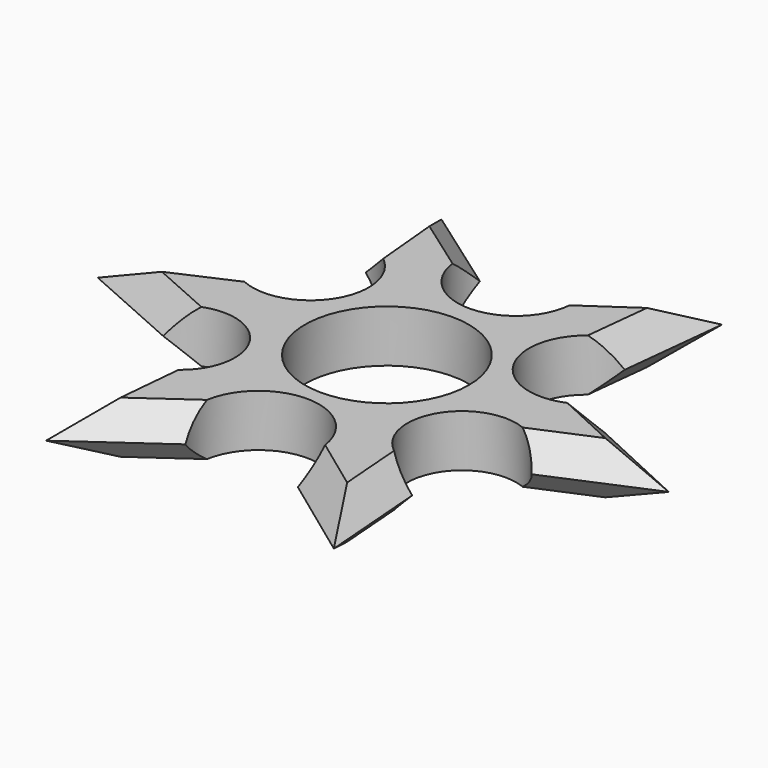
from build123d import *

# Parameters (mm, degrees)
F0_R         = 11
F1_DEPTH     = 7
F2_SIZE      = 3.81
F3_T1_DEPTH  = 34.6394313852
F3_T3_DEPTH  = 34.3439110976
F4_SIZE      = 3.81
F5_T1_DEPTH  = 35.2279158768
F5_T3_DEPTH  = 35.1515641575
F5_T5_DEPTH  = 34.8076073963
F5_T7_DEPTH  = 34.8076073963
F5_T9_DEPTH  = 34.5979192148
F5_T11_DEPTH = 35.1515641575
F5_T13_DEPTH = 35.2279158768
F5_T15_DEPTH = 34.6394313852
F5_T17_DEPTH = 34.8076073963
F6_T1_DEPTH  = 29.7856896268


# Not quite as in the source:
# - a fillet or chamfer that OpenCascade refuses, or shapes differently, is made with other operations: its cross-section is extruded or revolved along the edge and cut away or added


with BuildPart() as f1:
    # F0 (on Top) → F1 (new body)
    with BuildSketch(Plane.XY):
        with BuildLine():
            Line((-19.3098304855, 33.4750442975), (-17.9191186068, 18.4962593726))
            ThreePointArc((-17.9191186068, 18.4962593726), (-12.1734101316, 6.7065768921), (-25.2838117957, 6.35))
            Line((-25.2838117957, 6.35), (-39.5676235915, 0))
            Line((-39.5676235915, 0), (-25.3535799067, -6.3189839441))
            ThreePointArc((-25.3535799067, -6.3189839441), (-12.9763127609, -6.8724869317), (-18.8926645602, -17.7582523592))
            Line((-18.8926645602, -17.7582523592), (-20.2989239466, -32.9044930863))
            Line((-20.2989239466, -32.9044930863), (-7.891724267, -24.1040629982))
            ThreePointArc((-7.891724267, -24.1040629982), (-0.2207247048, -12.9944902326), (7.1436805269, -24.3096295115))
            Line((7.1436805269, -24.3096295115), (19.2464965418, -33.1737534264))
            Line((19.2464965418, -33.1737534264), (19.2872961226, -33.1740312262))
            Line((19.2872961226, -33.1740312262), (18.113880894, -18.0395493303))
            ThreePointArc((18.113880894, -18.0395493303), (12.3636945983, -7.0651033251), (24.7479456966, -6.6998194754))
            Line((24.7479456966, -6.6998194754), (39.056406052, -0.5976429607))
            Line((39.056406052, -0.5976429607), (24.8707754105, 5.9687611329))
            ThreePointArc((24.8707754105, 5.9687611329), (11.7673092468, 6.524596873), (17.6915767021, 18.225572644))
            Line((17.6915767021, 18.225572644), (19.3098304855, 33.1814855899))
            Line((19.3098304855, 33.1814855899), (7.1525325905, 24.8331700857))
            ThreePointArc((7.1525325905, 24.8331700857), (0.2505296838, 13.6219778067), (-6.9026308059, 24.6746142094))
            Line((-6.9026308059, 24.6746142094), (-19.3098304855, 33.4750442975))
        make_face()
        Circle(F0_R, mode=Mode.SUBTRACT)
    extrude(amount=F1_DEPTH)

    # F2
    f2_edges = [f1.edges().sort_by_distance(p)[0] for p in [
        (18.500704, 25.703529, 7),
        (13.231182, 29.007328, 7),
    ]]
    chamfer(f2_edges, length=F2_SIZE)

    # F3: chamfer of 3.81 on 2 edges, made by hand

    # F3_s2 → F3_t1 (cut)
    with BuildSketch(Plane(origin=(1.0999249917, 10.1655145758, 0), x_dir=(0, 0, 1), z_dir=(0.1075737229, 0.9941971103, 0))):
        Polygon((3.81, 15.6283217323), (0, 11.8183217323), (0, 15.6283217323), align=None)
    extrude(amount=F3_T1_DEPTH, mode=Mode.SUBTRACT)

    # F3_s4 → F3_t3 (cut)
    with BuildSketch(Plane(origin=(36.6832724438, 25.190098551, 0), x_dir=(0, 0, 1), z_dir=(-0.8243528709, -0.5660762706, 0))):
        Polygon((0, 12.6124160802), (3.81, 16.4224160802), (0, 16.4224160802), align=None)
    extrude(amount=F3_T3_DEPTH, mode=Mode.SUBTRACT)

    # F4 (call 1 of 6: OpenCascade refuses the feature's edges together)
    f4_edges = [f1.edges().sort_by_distance(p)[0] for p in [
        (31.902176, -3.648731, 7),
        (31.963591, 2.685559, 7),
    ]]
    chamfer(f4_edges, length=F4_SIZE)

    # F4#2 (call 2 of 6)
    f4_2_edges = [f1.edges().sort_by_distance(p)[0] for p in [
        (18.700589, -25.60679, 7),
    ]]
    chamfer(f4_2_edges, length=F4_SIZE)

    # F4#3 (call 3 of 6)
    f4_3_edges = [f1.edges().sort_by_distance(p)[0] for p in [
        (13.195089, -28.741691, 7),
    ]]
    chamfer(f4_3_edges, length=F4_SIZE)

    # F4#4 (call 4 of 6)
    f4_4_edges = [f1.edges().sort_by_distance(p)[0] for p in [
        (-14.095324, -28.504278, 7),
        (-19.595794, -25.331373, 7),
    ]]
    chamfer(f4_4_edges, length=F4_SIZE)

    # F4#5 (call 5 of 6)
    f4_5_edges = [f1.edges().sort_by_distance(p)[0] for p in [
        (-32.460602, -3.159492, 7),
        (-32.425718, 3.175, 7),
    ]]
    chamfer(f4_5_edges, length=F4_SIZE)

    # F4#6 (call 6 of 6)
    f4_6_edges = [f1.edges().sort_by_distance(p)[0] for p in [
        (-18.614475, 25.985652, 7),
        (-13.106231, 29.074829, 7),
    ]]
    chamfer(f4_6_edges, length=F4_SIZE)

    # F5: chamfer of 3.81 on 9 edges, made by hand

    # F5_s2 → F5_t1 (cut)
    with BuildSketch(Plane(origin=(41.2840936669, -19.1100451228, 0), x_dir=(0, 0, 1), z_dir=(-0.9074917218, 0.4200699643, 0))):
        Polygon((0, 12.0540670557), (3.81, 15.8640670557), (0, 15.8640670557), align=None)
    extrude(amount=F5_T1_DEPTH, mode=Mode.SUBTRACT)

    # F5_s4 → F5_t3 (cut)
    with BuildSketch(Plane(origin=(9.5091795604, 4.0554113263, 0), x_dir=(0, 0, 1), z_dir=(0.9198423531, 0.3922882173, 0))):
        Polygon((0, 12.0611052097), (3.81, 15.8711052097), (0, 15.8711052097), align=None)
    extrude(amount=F5_T3_DEPTH, mode=Mode.SUBTRACT)

    # F5_s6 → F5_t5 (cut)
    with BuildSketch(Plane(origin=(-37.0237803275, -26.260977399, 0), x_dir=(0, 0, 1), z_dir=(0.8156523083, 0.5785424029, 0))):
        Polygon((0, 11.2848375041), (3.81, 15.0948375041), (0, 15.0948375041), align=None)
    extrude(amount=F5_T5_DEPTH, mode=Mode.SUBTRACT)

    # F5_s8 → F5_t7 (cut)
    with BuildSketch(Plane(origin=(-0.8903351992, -9.5894337742, 0), x_dir=(0, 0, 1), z_dir=(-0.0924478322, -0.9957175294, 0))):
        Polygon((0, 13.3600453443), (3.81, 17.1700453443), (0, 17.1700453443), align=None)
    extrude(amount=F5_T7_DEPTH, mode=Mode.SUBTRACT)

    # F5_s10 → F5_t9 (cut)
    with BuildSketch(Plane(origin=(8.3331341524, -6.1032022329, 0), x_dir=(0, 0, 1), z_dir=(0.806763245, -0.5908748315, 0))):
        Polygon((0, 11.5810945617), (3.81, 15.3910945617), (0, 15.3910945617), align=None)
    extrude(amount=F5_T9_DEPTH, mode=Mode.SUBTRACT)

    # F5_s12 → F5_t11 (cut)
    with BuildSketch(Plane(origin=(-41.9914373351, 18.6676799506, 0), x_dir=(0, 0, 1), z_dir=(0.9137726258, -0.406226031, 0))):
        Polygon((0, 12.2633986894), (3.81, 16.0733986894), (0, 16.0733986894), align=None)
    extrude(amount=F5_T11_DEPTH, mode=Mode.SUBTRACT)

    # F5_s14 → F5_t13 (cut)
    with BuildSketch(Plane(origin=(-9.8011321421, -4.357183502, 0), x_dir=(0, 0, 1), z_dir=(-0.9137726258, -0.406226031, 0))):
        Polygon((3.81, 16.0733986894), (0, 12.2633986894), (0, 16.0733986894), align=None)
    extrude(amount=F5_T13_DEPTH, mode=Mode.SUBTRACT)

    # F5_s16 → F5_t15 (cut)
    with BuildSketch(Plane(origin=(-4.1522899993, 44.7226055925, 0), x_dir=(0, 0, 1), z_dir=(0.0924478322, -0.9957175294, 0))):
        Polygon((3.81, 16.1324414242), (0, 12.3224414242), (0, 16.1324414242), align=None)
    extrude(amount=F5_T15_DEPTH, mode=Mode.SUBTRACT)

    # F5_s18 → F5_t17 (cut)
    with BuildSketch(Plane(origin=(-8.2440794116, 5.8475277562, 0), x_dir=(0, 0, 1), z_dir=(-0.8156523083, 0.5785424029, 0))):
        Polygon((0, 12.3224414242), (3.81, 16.1324414242), (0, 16.1324414242), align=None)
    extrude(amount=F5_T17_DEPTH, mode=Mode.SUBTRACT)

    # F6: chamfer of 3.81 on 1 edges, made by hand

    # F6_s2 → F6_t1 (cut)
    with BuildSketch(Plane(origin=(3.0435836487, -39.2555512393, 0), x_dir=(0, 0, 1), z_dir=(-0.0773005765, 0.9970078339, 0))):
        Polygon((0, 12.8552135911), (3.81, 16.6652135911), (0, 16.6652135911), align=None)
    extrude(amount=F6_T1_DEPTH, mode=Mode.SUBTRACT)


solid = f1.part
